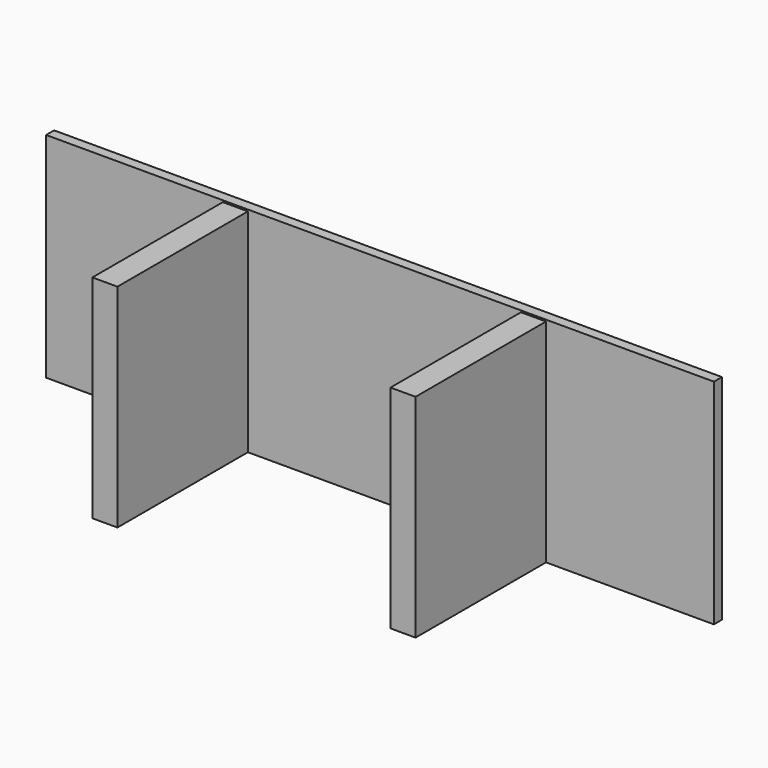
from build123d import *

# Parameters (mm, degrees)
F0_W     = 8.9696688134
F0_H     = 6
F0_W_2   = 6.0303311866
F0_W_3   = 7.6489803101
F0_W_4   = 7.3510196899
F2_DEPTH = 128
F4_DEPTH = 127


# Not quite as in the source:
# - the program builds the solid bodies; features that only make, move or delete a surface that nothing else refers to are left out


with BuildPart() as f2:
    # F0 (on Top) → F2 (new body)
    with BuildSketch(Plane.XY):
        Polygon((-400, 0), (-294.1345971149, 0), (-294.1345971149, 6), (-299.6463162062, 6), (-311.9468285562, 6), (-322.7511938045, 6), (-335.9566328529, 6), (-348.7171674377, 6), (-362.4063217106, 6), (-376.9397732412, 6), (-400, 6), align=None)
        with Locations((-283.6194315216, 3)):
            Rectangle(F0_W, F0_H)
        with Locations((-291.1194315216, 3)):
            Rectangle(F0_W_2, F0_H)
        Polygon((-279.1345971149, 0), (-115.5724730993, 0), (-115.5724730993, 6), (-120.0142995768, 6), (-130.6865749399, 6), (-142.439753188, 6), (-152.7159749868, 6), (-164.8405666594, 6), (-175.9109262937, 6), (-188.4297876225, 6), (-205.2331021726, 6), (-216.1265840576, 6), (-227.5328489064, 6), (-240.1054796123, 6), (-251.4180912129, 6), (-260.7190593146, 6), (-272.6732546984, 6), (-279.1345971149, 6), align=None)
        with Locations((-111.7479829443, 3)):
            Rectangle(F0_W_3, F0_H)
        with Locations((-104.2479829443, 3)):
            Rectangle(F0_W_4, F0_H)
        Polygon((-100.5724730993, 0), (0, 0), (0, 6), (-21.7185619105, 6), (-32.3376952831, 6), (-47.4983571934, 6), (-60.9528624883, 6), (-73.3657559167, 6), (-83.3882540464, 6), (-97.7746488723, 6), (-100.5724730993, 6), align=None)
    extrude(amount=F2_DEPTH)

    # F0 (on Top) → F4 (join)
    with BuildSketch(Plane.XY):
        Polygon((-279.1345971149, -97.6634095667), (-279.1345971149, 0), (-288.1042659283, 0), (-294.1345971149, 0), (-294.1345971149, -97.6634095667), align=None)
        Polygon((-100.5724730993, -97.6634095667), (-100.5724730993, 0), (-107.9234927893, 0), (-115.5724730993, 0), (-115.5724730993, -97.6634095667), align=None)
    extrude(amount=F4_DEPTH)


solid = f2.part
